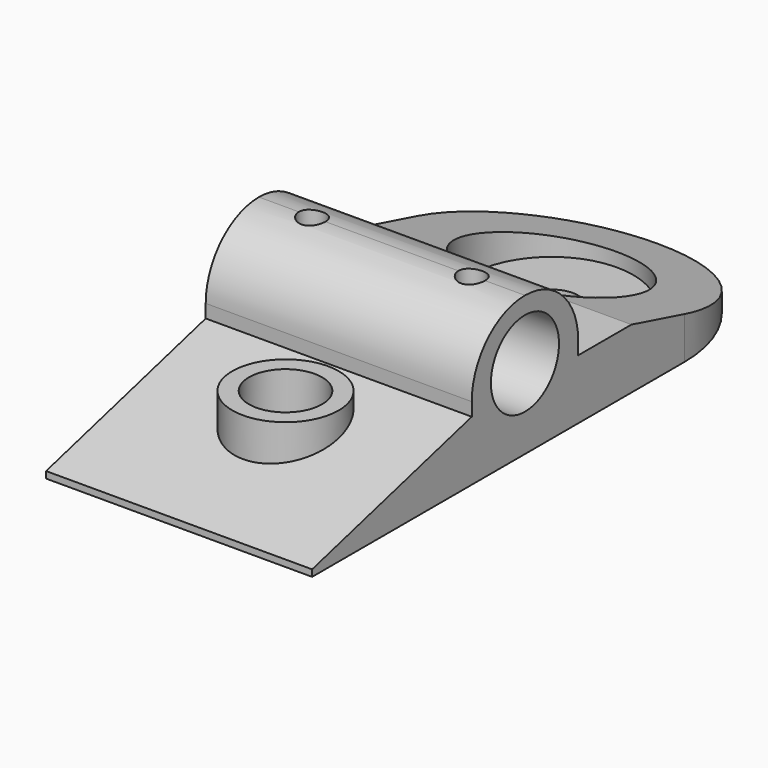
from build123d import *

# Parameters (mm, degrees)
F0_W         = 20
F0_H         = 45
F0_R         = 4
F0_R_2       = 6.15
F1_DEPTH     = 4
F1_FACE_W    = 20
F1_FACE_H    = 45
F1_FACE_R    = 4
F1_FACE_R_2  = 6.15
F0_R_3       = 2
F0_R_4       = 2.75
F2_DEPTH     = 0.5
F4_T1_DEPTH  = 97.9025398997
F5_DEPTH     = 5
F3_W         = 20
F3_H         = 10
F6_DEPTH     = 6
F7_R         = 3.2
F8_DEPTH     = 25
F10_R        = 9.99999
F11_R        = 1
F12_DEPTH    = 25
F13_T1_DEPTH = 45


# Not quite as in the source:
# - a fillet or chamfer that OpenCascade refuses, or shapes differently, is made with other operations: its cross-section is extruded or revolved along the edge and cut away or added
# - a fillet or chamfer is up to 0.001 mm smaller than in the source, because OpenCascade refuses the exact size
# - a feature of the source that left no trace in its solid (it failed there, or was rolled back) is left out


with BuildPart() as f1:
    # F0 (on Top) → F1 (new body)
    with BuildSketch(Plane.XY):
        with Locations((10, 22.5)):
            Rectangle(F0_W, F0_H)
        with Locations((10, 10)):
            Circle(F0_R, mode=Mode.SUBTRACT)
        with Locations((10, 35)):
            Circle(F0_R_2, mode=Mode.SUBTRACT)
    extrude(amount=F1_DEPTH)

    # F1_face (on face) + F0 (on Top) → F2 (join)
    with BuildSketch(Plane(origin=(10, 21.3275360022, 4), x_dir=(1, 0, 0), z_dir=(0, 0, 1))):
        with Locations((0, 1.1724639978)):
            Rectangle(F1_FACE_W, F1_FACE_H)
        with Locations((0, -11.3275360022)):
            Circle(F1_FACE_R, mode=Mode.SUBTRACT)
        with Locations((0, 13.6724639978)):
            Circle(F1_FACE_R_2, mode=Mode.SUBTRACT)
    with BuildSketch(Plane.XY):
        with Locations((10, 35)):
            Circle(F0_R_2)
        with Locations((10, 35)):
            Circle(F0_R_3, mode=Mode.SUBTRACT)
        with Locations((10, 10)):
            Circle(F0_R_4)
    extrude(amount=F2_DEPTH)

    # F4: chamfer of 15 x 4 on 2 edges, made by hand

    # F4_s2 → F4_t1 (cut)
    with BuildSketch(Plane.YZ.offset(-38.9512699498)):
        Polygon((0, 0.5), (15, 4.5), (0, 4.5), align=None)
        Polygon((30, 4.5), (45, 0.5), (45, 4.5), align=None)
    extrude(amount=F4_T1_DEPTH, mode=Mode.SUBTRACT)

    # F0 (on Top) → F5 (join)
    with BuildSketch(Plane.XY):
        with Locations((10, 10)):
            Circle(F0_R)
        with Locations((10, 10)):
            Circle(F0_R_4, mode=Mode.SUBTRACT)
    extrude(amount=F5_DEPTH)

    # F3 (on face) → F6 (join)
    with BuildSketch(Plane.XY.offset(4.5)):
        with Locations((10, 20)):
            Rectangle(F3_W, F3_H)
    extrude(amount=F6_DEPTH)

    # F7 (on face) → F8 (cut)
    with BuildSketch(Plane(origin=(0, 0, 0), x_dir=(0, -1, 0), z_dir=(-1, 0, 0))):
        with Locations((-20, 6)):
            Circle(F7_R)
    extrude(amount=-F8_DEPTH, mode=Mode.SUBTRACT)

    # F10 (radius 10 in the source; OpenCascade refuses exactly that, so slightly less here)
    f10_edges = [f1.edges().sort_by_distance(p)[0] for p in [
        (0, 45, 0.25),
        (20, 45, 0.25),
    ]]
    fillet(f10_edges, radius=F10_R)

    # F11 (on face) → F12 (cut)
    with BuildSketch(Plane.XY.offset(10.5)):
        with Locations((4, 20)):
            Circle(F11_R)
        with Locations((16, 20)):
            Circle(F11_R)
    extrude(amount=-F12_DEPTH, mode=Mode.SUBTRACT)

    # F13: fillet of radius 5 on 2 edges, made by hand

    # F13_s2 → F13_t1 (cut)
    with BuildSketch(Plane.YZ.offset(-12.5)):
        with BuildLine():
            ThreePointArc((25, 5.5), (23.5355339059, 9.0355339059), (20, 10.5))
            Line((20, 10.5), (25, 10.5))
            Line((25, 10.5), (25, 5.5))
        make_face()
        with BuildLine():
            ThreePointArc((20, 10.5), (16.4644660941, 9.0355339059), (15, 5.5))
            Line((15, 5.5), (15, 10.5))
            Line((15, 10.5), (20, 10.5))
        make_face()
    extrude(amount=F13_T1_DEPTH, mode=Mode.SUBTRACT)


solid = f1.part
